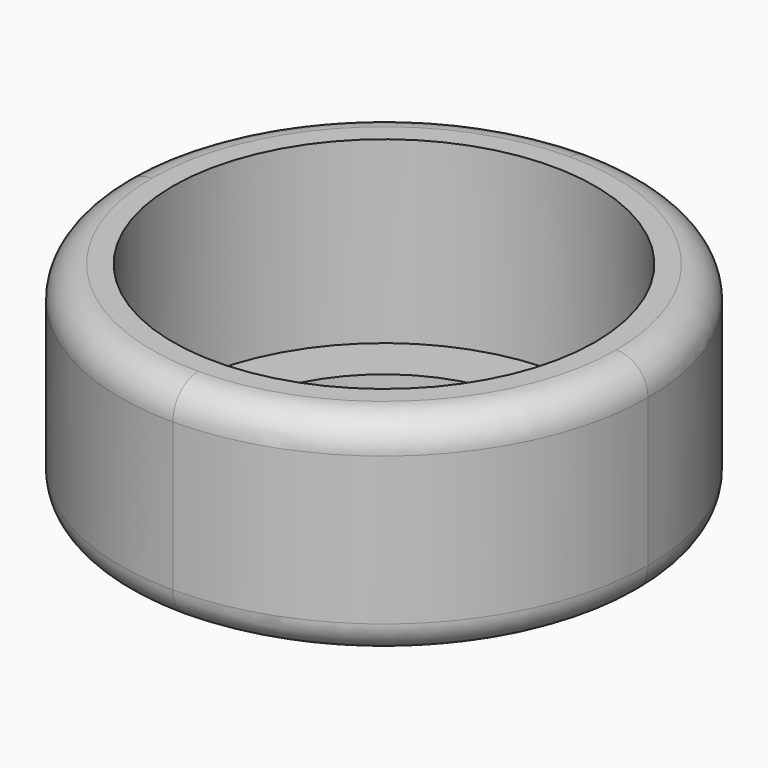
from build123d import *

# Parameters (mm, degrees)
F0_W     = 50
F0_H     = 50
F0_R     = 15
F1_DEPTH = 20
F2_R     = 20
F3_DEPTH = 20
F6_R     = 24.99999
F7_R     = 3


# Not quite as in the source:
# - a fillet or chamfer is up to 0.001 mm smaller than in the source, because OpenCascade refuses the exact size


with BuildPart() as f1:
    # F0 (on Top) → F1 (new body)
    with BuildSketch(Plane.XY):
        Rectangle(F0_W, F0_H)
        Circle(F0_R, mode=Mode.SUBTRACT)
    extrude(amount=F1_DEPTH)


with BuildPart() as f3:
    # F2 (on Top) → F3 (new body)
    with BuildSketch(Plane.XY):
        Circle(F2_R)
    extrude(amount=F3_DEPTH)


with BuildPart() as f3_1:
    # F4: moved
    add(f3.part.moved(Location((0, 0, 3))))


with BuildPart() as f1_1:
    add(f1.part)

    # F5: cut F3
    add(f3_1.part, mode=Mode.SUBTRACT)

    # F6 (radius 25 in the source; OpenCascade refuses exactly that, so slightly less here)
    f6_edges = [f1_1.edges().sort_by_distance(p)[0] for p in [
        (-25, 25, 10),
        (-25, -25, 10),
        (25, -25, 10),
        (25, 25, 10),
    ]]
    fillet(f6_edges, radius=F6_R)

    # F7
    f7_edges = [f1_1.edges().sort_by_distance(p)[0] for p in [
        (-17.677672, 17.677672, 0),
        (-17.677672, 17.677672, 20),
    ]]
    fillet(f7_edges, radius=F7_R)


solid = f1_1.part
